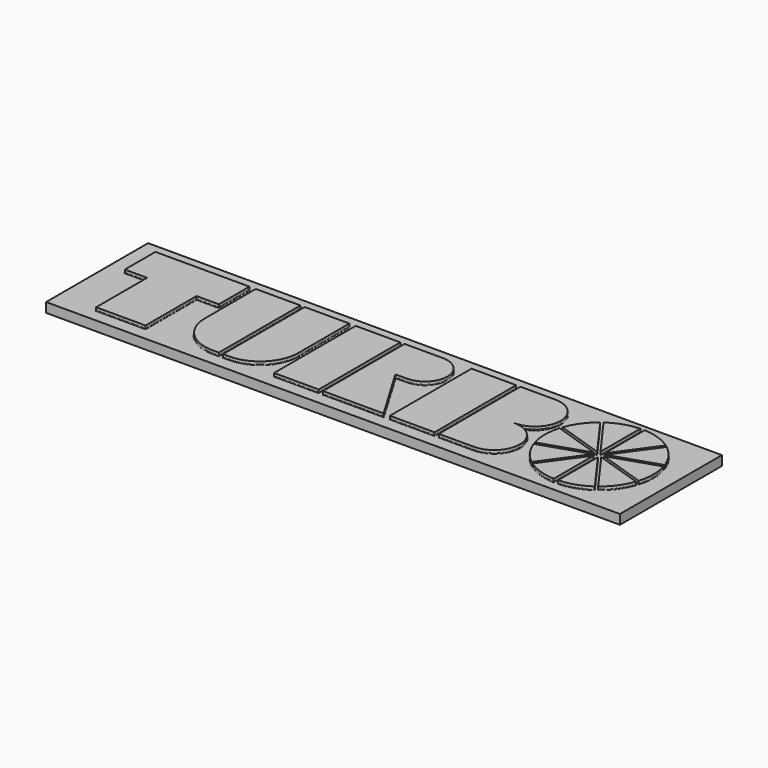
from build123d import *

# Parameters (mm, degrees)
F1_DEPTH = 2
F0_W     = 7
F0_H     = 16
F3_W     = 90
F3_H     = 20
F4_DEPTH = 1.5
F8_ANGLE = 180
F9_R     = 0.1
F12_R    = 0.1


# Not quite as in the source:
# - a feature names something its author has since deleted; it is built from what else it names


with BuildPart() as f1:
    # F0 (on Top) → F1 (new body)
    with BuildSketch(Plane.XY):
        Polygon((-35.3233079513, -13.3071839809), (-20.5771312745, -13.3071839809), (-20.5771312745, -7.3071839809), (-24.0771312745, -7.3071839809), (-24.0771312745, 2.6928160191), (-31.8233079513, 2.6928160191), (-31.8233079513, -7.3071839809), (-35.3233079513, -7.3071839809), align=None)
    extrude(amount=F1_DEPTH)


with BuildPart() as f1b:
    # F0 (on Top) → F1, piece 2 (new body)
    with BuildSketch(Plane.XY):
        with BuildLine():
            Line((-19.5771312745, -3.3071839809), (-19.5771312745, -13.3071839809))
            Line((-19.5771312745, -13.3071839809), (-12.5771312745, -13.3071839809))
            Line((-12.5771312745, -13.3071839809), (-12.5771312745, 2.6928160191))
            Line((-12.5771312745, 2.6928160191), (-13.5771312745, 2.6928160191))
            ThreePointArc((-13.5771312745, 2.6928160191), (-17.8197719616, 0.9354567062), (-19.5771312745, -3.3071839809))
        make_face()
    extrude(amount=F1_DEPTH)


with BuildPart() as f1c:
    # F0 (on Top) → F1, piece 3 (new body)
    with BuildSketch(Plane.XY):
        with BuildLine():
            Line((-11.9104646078, 2.6928160191), (-11.9104646078, -13.3071839809))
            Line((-11.9104646078, -13.3071839809), (-4.9104646078, -13.3071839809))
            Line((-4.9104646078, -13.3071839809), (-4.9104646078, -3.3071839809))
            ThreePointArc((-4.9104646078, -3.3071839809), (-6.6678239207, 0.9354567062), (-10.9104646078, 2.6928160191))
            Line((-10.9104646078, 2.6928160191), (-11.9104646078, 2.6928160191))
        make_face()
    extrude(amount=F1_DEPTH)


with BuildPart() as f1d:
    # F0 (on Top) → F1, piece 4 (new body)
    with BuildSketch(Plane.XY):
        with Locations((-0.4104646078, -5.3071839809)):
            Rectangle(F0_W, F0_H)
    extrude(amount=F1_DEPTH)


with BuildPart() as f1e:
    # F0 (on Top) → F1, piece 5 (new body)
    with BuildSketch(Plane.XY):
        with BuildLine():
            Line((3.7562020589, -6.3071839809), (3.7562020589, -13.3071839809))
            Line((3.7562020589, -13.3071839809), (9.7562020589, -13.3071839809))
            ThreePointArc((9.7562020589, -13.3071839809), (12.231075793, -12.2820577151), (13.2562020589, -9.8071839809))
            ThreePointArc((13.2562020589, -9.8071839809), (12.231075793, -7.3323102468), (9.7562020589, -6.3071839809))
            Line((9.7562020589, -6.3071839809), (7.9124520589, -6.3071839809))
            Line((7.9124520589, -6.3071839809), (13.2562020589, 2.6928160191))
            Line((13.2562020589, 2.6928160191), (3.7562020589, 2.6928160191))
            Line((3.7562020589, 2.6928160191), (3.7562020589, -6.3071839809))
        make_face()
    extrude(amount=F1_DEPTH)


with BuildPart() as f1f:
    # F0 (on Top) → F1, piece 6 (new body)
    with BuildSketch(Plane.XY):
        with Locations((17.7562020589, -5.3071839809)):
            Rectangle(F0_W, F0_H)
    extrude(amount=F1_DEPTH)


with BuildPart() as f1g:
    # F0 (on Top) → F1, piece 7 (new body)
    with BuildSketch(Plane.XY):
        with BuildLine():
            Line((21.9228687255, -5.3071839809), (21.9228687255, -13.3071839809))
            Line((21.9228687255, -13.3071839809), (27.4228687255, -13.3071839809))
            ThreePointArc((27.4228687255, -13.3071839809), (30.2512958503, -12.1356111057), (31.4228687255, -9.3071839809))
            ThreePointArc((31.4228687255, -9.3071839809), (30.2512958503, -6.4787568562), (27.4228687255, -5.3071839809))
            ThreePointArc((27.4228687255, -5.3071839809), (30.2512958503, -4.1356111057), (31.4228687255, -1.3071839809))
            ThreePointArc((31.4228687255, -1.3071839809), (30.2512958503, 1.5212431438), (27.4228687255, 2.6928160191))
            Line((27.4228687255, 2.6928160191), (21.9228687255, 2.6928160191))
            Line((21.9228687255, 2.6928160191), (21.9228687255, -5.3071839809))
        make_face()
    extrude(amount=F1_DEPTH)


with BuildPart() as f1h:
    # F0 (on Top) → F1, piece 8 (new body)
    with BuildSketch(Plane.XY):
        with BuildLine():
            Line((35.7953587214, 1.6514498611), (40.3433587154, -4.6353291686))
            Line((40.3433587154, -4.6353291686), (40.3433587154, 3.1862775566))
            ThreePointArc((40.3433587154, 3.1862775566), (37.9587680047, 2.7465660084), (35.7953587214, 1.6514498611))
        make_face()
    extrude(amount=F1_DEPTH)


with BuildPart() as f1i:
    # F0 (on Top) → F1, piece 9 (new body)
    with BuildSketch(Plane.XY):
        with BuildLine():
            Line((32.6585957081, -2.4858135563), (40.0384314777, -4.9133268451))
            Line((40.0384314777, -4.9133268451), (35.4654683426, 1.4079591661))
            ThreePointArc((35.4654683426, 1.4079591661), (33.7814695195, -0.3366803573), (32.6585957081, -2.4858135563))
        make_face()
    extrude(amount=F1_DEPTH)


with BuildPart() as f1j:
    # F0 (on Top) → F1, piece 10 (new body)
    with BuildSketch(Plane.XY):
        with BuildLine():
            Line((32.5290165176, -7.7290393525), (39.8916517633, -5.3071839809))
            Line((39.8916517633, -5.3071839809), (32.5290165176, -2.8853286094))
            ThreePointArc((32.5290165176, -2.8853286094), (32.1766920487, -5.3071839809), (32.5290165176, -7.7290393525))
        make_face()
    extrude(amount=F1_DEPTH)


with BuildPart() as f1k:
    # F0 (on Top) → F1, piece 11 (new body)
    with BuildSketch(Plane.XY):
        with BuildLine():
            Line((35.4654683426, -12.022327128), (40.0384314777, -5.7010411168))
            Line((40.0384314777, -5.7010411168), (32.6585957081, -8.1285544056))
            ThreePointArc((32.6585957081, -8.1285544056), (33.7814695195, -10.2776876045), (35.4654683426, -12.022327128))
        make_face()
    extrude(amount=F1_DEPTH)


with BuildPart() as f1l:
    # F0 (on Top) → F1, piece 12 (new body)
    with BuildSketch(Plane.XY):
        with BuildLine():
            ThreePointArc((35.7953587214, -12.265817823), (37.9587680047, -13.3609339703), (40.3433587154, -13.8006455184))
            Line((40.3433587154, -13.8006455184), (40.3433587154, -5.9790387933))
            Line((40.3433587154, -5.9790387933), (35.7953587214, -12.265817823))
        make_face()
    extrude(amount=F1_DEPTH)


with BuildPart() as f1m:
    # F0 (on Top) → F1, piece 13 (new body)
    with BuildSketch(Plane.XY):
        with BuildLine():
            Line((41.010025382, -5.9790387933), (41.010025382, -13.8006455184))
            ThreePointArc((41.010025382, -13.8006455184), (43.3946160927, -13.3609339703), (45.558025376, -12.265817823))
            Line((45.558025376, -12.265817823), (41.010025382, -5.9790387933))
        make_face()
    extrude(amount=F1_DEPTH)


with BuildPart() as f1n:
    # F0 (on Top) → F1, piece 14 (new body)
    with BuildSketch(Plane.XY):
        with BuildLine():
            Line((41.3149526198, -5.7010411168), (45.8879157548, -12.022327128))
            ThreePointArc((45.8879157548, -12.022327128), (47.5719145779, -10.2776876045), (48.6947883893, -8.1285544056))
            Line((48.6947883893, -8.1285544056), (41.3149526198, -5.7010411168))
        make_face()
    extrude(amount=F1_DEPTH)


with BuildPart() as f1o:
    # F0 (on Top) → F1, piece 15 (new body)
    with BuildSketch(Plane.XY):
        with BuildLine():
            Line((48.8212399464, -2.8748313044), (41.4266920487, -5.3071839809))
            Line((41.4266920487, -5.3071839809), (48.8212399464, -7.7395366574))
            ThreePointArc((48.8212399464, -7.7395366574), (49.1766920487, -5.3071839809), (48.8212399464, -2.8748313044))
        make_face()
    extrude(amount=F1_DEPTH)


with BuildPart() as f1p:
    # F0 (on Top) → F1, piece 16 (new body)
    with BuildSketch(Plane.XY):
        with BuildLine():
            Line((45.8879157548, 1.4079591661), (41.3149526198, -4.9133268451))
            Line((41.3149526198, -4.9133268451), (48.6947883893, -2.4858135563))
            ThreePointArc((48.6947883893, -2.4858135563), (47.5719145779, -0.3366803573), (45.8879157548, 1.4079591661))
        make_face()
    extrude(amount=F1_DEPTH)


with BuildPart() as f1q:
    # F0 (on Top) → F1, piece 17 (new body)
    with BuildSketch(Plane.XY):
        with BuildLine():
            Line((41.010025382, 3.1862775566), (41.010025382, -4.6353291686))
            Line((41.010025382, -4.6353291686), (45.558025376, 1.6514498611))
            ThreePointArc((45.558025376, 1.6514498611), (43.3946160927, 2.7465660084), (41.010025382, 3.1862775566))
        make_face()
    extrude(amount=F1_DEPTH)


with BuildPart() as f4:
    # F3 (on offset) → F4 (new body)
    with BuildSketch(Plane.XY.offset(2)):
        with Locations((6.9266920487, -5.3071839809)):
            Rectangle(F3_W, F3_H)
    extrude(amount=-F4_DEPTH)


with BuildPart() as f1_1:
    # F5: moved
    add(f1.part)


with BuildPart() as f1b_1:
    # F5: moved
    add(f1b.part)


with BuildPart() as f1c_1:
    # F5: moved
    add(f1c.part)


with BuildPart() as f1d_1:
    # F5: moved
    add(f1d.part)


with BuildPart() as f1e_1:
    # F5: moved
    add(f1e.part)


with BuildPart() as f1f_1:
    # F5: moved
    add(f1f.part)


with BuildPart() as f1g_1:
    # F5: moved
    add(f1g.part)


with BuildPart() as f1m_1:
    # F5: moved
    add(f1m.part)


with BuildPart() as f1l_1:
    # F5: moved
    add(f1l.part)


with BuildPart() as f1h_1:
    # F5: moved
    add(f1h.part)


with BuildPart() as f1q_1:
    # F5: moved
    add(f1q.part)


with BuildPart() as f1p_1:
    # F5: moved
    add(f1p.part)


with BuildPart() as f1i_1:
    # F5: moved
    add(f1i.part)


with BuildPart() as f1n_1:
    # F5: moved
    add(f1n.part)


with BuildPart() as f1k_1:
    # F5: moved
    add(f1k.part)


with BuildPart() as f1o_1:
    # F5: moved
    add(f1o.part)


with BuildPart() as f1j_1:
    # F5: moved
    add(f1j.part)


with BuildPart() as f4_1:
    # F5: moved
    add(f4.part)


with BuildPart() as f1_2:
    # F6: moved
    add(f1_1.part.moved(Location((-3.1, -2.4, 9.9))))


with BuildPart() as f1b_2:
    # F6: moved
    add(f1b_1.part.moved(Location((-3.1, -2.4, 9.9))))


with BuildPart() as f1c_2:
    # F6: moved
    add(f1c_1.part.moved(Location((-3.1, -2.4, 9.9))))


with BuildPart() as f1d_2:
    # F6: moved
    add(f1d_1.part.moved(Location((-3.1, -2.4, 9.9))))


with BuildPart() as f1e_2:
    # F6: moved
    add(f1e_1.part.moved(Location((-3.1, -2.4, 9.9))))


with BuildPart() as f1f_2:
    # F6: moved
    add(f1f_1.part.moved(Location((-3.1, -2.4, 9.9))))


with BuildPart() as f1g_2:
    # F6: moved
    add(f1g_1.part.moved(Location((-3.1, -2.4, 9.9))))


with BuildPart() as f1m_2:
    # F6: moved
    add(f1m_1.part.moved(Location((-3.1, -2.4, 9.9))))


with BuildPart() as f1l_2:
    # F6: moved
    add(f1l_1.part.moved(Location((-3.1, -2.4, 9.9))))


with BuildPart() as f1h_2:
    # F6: moved
    add(f1h_1.part.moved(Location((-3.1, -2.4, 9.9))))


with BuildPart() as f1q_2:
    # F6: moved
    add(f1q_1.part.moved(Location((-3.1, -2.4, 9.9))))


with BuildPart() as f1p_2:
    # F6: moved
    add(f1p_1.part.moved(Location((-3.1, -2.4, 9.9))))


with BuildPart() as f1i_2:
    # F6: moved
    add(f1i_1.part.moved(Location((-3.1, -2.4, 9.9))))


with BuildPart() as f1n_2:
    # F6: moved
    add(f1n_1.part.moved(Location((-3.1, -2.4, 9.9))))


with BuildPart() as f1k_2:
    # F6: moved
    add(f1k_1.part.moved(Location((-3.1, -2.4, 9.9))))


with BuildPart() as f1o_2:
    # F6: moved
    add(f1o_1.part.moved(Location((-3.1, -2.4, 9.9))))


with BuildPart() as f1j_2:
    # F6: moved
    add(f1j_1.part.moved(Location((-3.1, -2.4, 9.9))))


with BuildPart() as f4_2:
    # F6: moved
    add(f4_1.part.moved(Location((-3.1, -2.4, 9.9))))


with BuildPart() as f1_3:
    add(f1_2.part)

    # F7: union F1b, F1c, F1d, F1e, F1f, F1g, F1m, F1l, F1h, F1q, F1p, F1i, F1n, F1k, F1o, F1j, F4
    add(f1b_2.part)
    add(f1c_2.part)
    add(f1d_2.part)
    add(f1e_2.part)
    add(f1f_2.part)
    add(f1g_2.part)
    add(f1m_2.part)
    add(f1l_2.part)
    add(f1h_2.part)
    add(f1q_2.part)
    add(f1p_2.part)
    add(f1i_2.part)
    add(f1n_2.part)
    add(f1k_2.part)
    add(f1o_2.part)
    add(f1j_2.part)
    add(f4_2.part)


with BuildPart() as f1_4:
    # F8: moved
    add(f1_3.part.rotate(Axis((3.8266920487, 2.2928160191, 11.9), (1, 0, 0)), F8_ANGLE))

    # F9
    f9_edges = [f1_4.edges().sort_by_distance(p)[0] for p in [
        (-34.923308, 9.292816, 13.4),
        (-36.673308, 14.292816, 13.4),
        (-38.423308, 17.292816, 13.4),
        (-31.05022, 4.292816, 13.4),
        (-27.177131, 9.292816, 13.4),
        (-25.427131, 14.292816, 13.4),
        (-31.05022, 20.292816, 13.4),
        (-23.677131, 17.292816, 13.4),
        (-20.919772, 6.050175, 13.4),
        (-9.767824, 6.050175, 13.4),
        (-14.510465, 4.292816, 13.4),
        (-16.177131, 4.292816, 13.4),
        (-8.010465, 15.292816, 13.4),
        (-11.510465, 20.292816, 13.4),
        (-19.177131, 20.292816, 13.4),
        (-15.677131, 12.292816, 13.4),
        (-15.010465, 12.292816, 13.4),
        (-7.010465, 12.292816, 13.4),
        (0.656202, 12.292816, 13.4),
        (-3.510465, 20.292816, 13.4),
        (-3.510465, 4.292816, 13.4),
        (5.406202, 4.292816, 13.4),
        (3.656202, 20.292816, 13.4),
        (10.156202, 16.792816, 13.4),
        (7.484327, 8.792816, 13.4),
    ]]
    fillet(f9_edges, radius=F9_R)


with BuildPart() as f1_5:
    # F10: moved
    add(f1_4.part.moved(Location((0, 0, -13.1))))


with BuildPart() as f1_6:
    # F11: moved
    add(f1_5.part.moved(Location((0, -10, 0))))

    # F12
    f12_edges = [f1_6.edges().sort_by_distance(p)[0] for p in [
        (14.656202, -5.707184, 0.3),
        (11.156202, 2.292816, 0.3),
        (21.572869, -5.707184, 0.3),
        (28.322869, -1.707184, 0.3),
        (18.822869, 2.292816, 0.3),
        (30.68147, -2.677688, 0.3),
        (29.076692, 2.292816, 0.3),
        (28.322869, 6.292816, 0.3),
        (30.68147, 7.26332, 0.3),
        (34.858768, -5.760934, 0.3),
        (14.656202, 10.292816, 0.3),
        (21.572869, 10.292816, 0.3),
        (34.858768, 10.346566, 0.3),
        (40.294616, 10.346566, 0.3),
        (40.294616, -5.760934, 0.3),
        (44.471915, -2.677688, 0.3),
        (46.076692, 2.292816, 0.3),
        (44.471915, 7.26332, 0.3),
        (18.156202, 2.292816, 0.3),
    ]]
    fillet(f12_edges, radius=F12_R)


solid = f1_6.part
